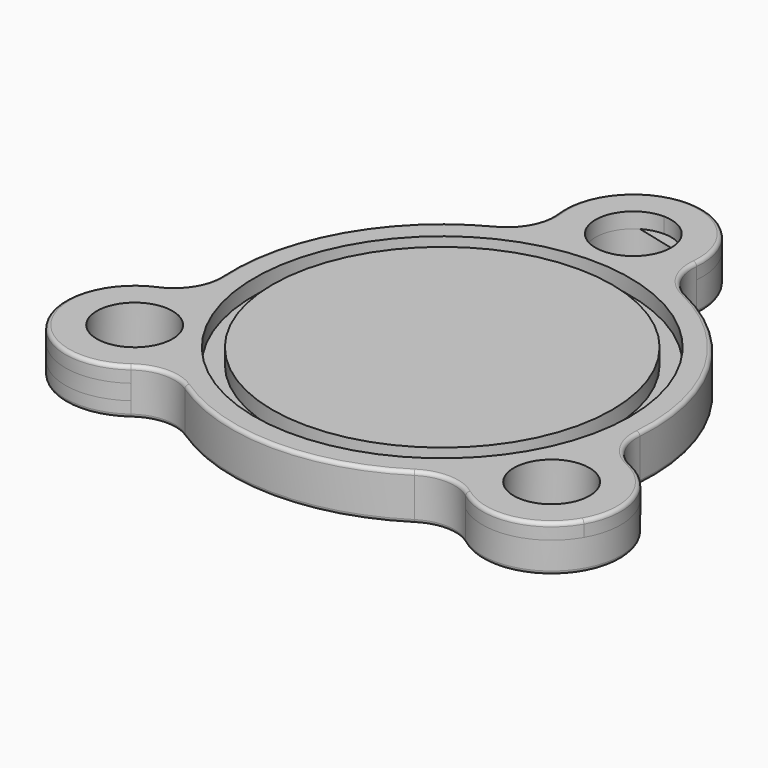
from build123d import *
from build123d import SkipClean  # not in build123d's __all__

# Parameters (mm, degrees)
F0_R     = 23.368
F2_DEPTH = 2.116667
F0_R_2   = 5.207
F0_R_3   = 25.8445
F3_R     = 5.207
F3_R_2   = 25.8445
F4_DEPTH = 2.116667
F5_R     = 5.207
F5_R_2   = 25.8445
F5_R_3   = 23.368
F6_DEPTH = 2.116667
F7_R     = 0.508


# Not quite as in the source:
# - after a boolean that leaves OpenCascade's solid faulty, fix() repairs it


with BuildPart() as f2:
    # F0 (on Top) → F2 (new body)
    with BuildSketch(Plane.XY):
        Circle(F0_R)
    extrude(amount=F2_DEPTH)



with BuildPart() as f2b:
    # F0 (on Top) → F2, piece 2 (new body)
    with BuildSketch(Plane.XY):
        with BuildLine():
            ThreePointArc((9.008634, 32.510164), (6.645647, 39.794521), (-0.316137, 42.984994))
            ThreePointArc((-0.316137, 42.984994), (-7.570395, 39.808854), (-9.915807, 32.245047))
            ThreePointArc((-9.915807, 32.245047), (-10.591058, 28.483521), (-13.302911, 25.790772))
            ThreePointArc((-13.302911, 25.790772), (-25.198767, 14.392829), (-28.972894, -1.644018))
            ThreePointArc((-28.972894, -1.644018), (-29.91458, -5.347837), (-32.811495, -7.840411))
            ThreePointArc((-32.811495, -7.840411), (-37.330955, -21.318933), (-23.425751, -24.275512))
            ThreePointArc((-23.425751, -24.275512), (-19.806913, -23.047075), (-16.138408, -24.118109))
            ThreePointArc((-16.138408, -24.118109), (-0.263504, -29.018304), (15.697768, -24.407201))
            ThreePointArc((15.697768, -24.407201), (19.385118, -23.402963), (22.981051, -24.696914))
            ThreePointArc((22.981051, -24.696914), (30.627799, -26.459145), (37.002427, -21.882867))
            ThreePointArc((37.002427, -21.882867), (37.818424, -14.195745), (32.663705, -8.434966))
            ThreePointArc((32.663705, -8.434966), (29.812532, -5.890196), (28.938261, -2.169887))
            ThreePointArc((28.938261, -2.169887), (25.127534, 14.516832), (12.575213, 26.153306))
            ThreePointArc((12.575213, 26.153306), (9.788992, 28.76903), (9.008634, 32.510164))
        make_face()
        with Locations((-29.059695, -16.595388)):
            Circle(F0_R_2, mode=Mode.SUBTRACT)
        with Locations((28.753535, -17.120367)):
            Circle(F0_R_2, mode=Mode.SUBTRACT)
        Circle(F0_R_3, mode=Mode.SUBTRACT)
        with BuildLine():
            ThreePointArc((4.738233, 33.461217), (-4.180055, 29.80893), (-0.385329, 38.667548))
            ThreePointArc((-0.385329, 38.667548), (3.24252, 37.113503), (4.738233, 33.461217))
        make_face(mode=Mode.SUBTRACT)
    extrude(amount=F2_DEPTH)


with BuildPart() as f2_1:
    add(f2.part, clean=False)

    with SkipClean():  # cleaning this boolean's faces spoils the solid; the shape is the same uncleaned
        add(f2b.part)  # F4 merges F2b
    # F3 (on face) → F4 (join)
    with BuildSketch(Plane(origin=(0, 0, 0), x_dir=(1, 0, 0), z_dir=(0, 0, -1))):
        with BuildLine():
            ThreePointArc((-13.302911, -25.790772), (-10.591058, -28.483521), (-9.915807, -32.245047))
            ThreePointArc((-9.915807, -32.245047), (-0.602192, -42.985282), (9.008634, -32.510164))
            ThreePointArc((9.008634, -32.510164), (9.788992, -28.76903), (12.575213, -26.153306))
            ThreePointArc((12.575213, -26.153306), (25.127534, -14.516832), (28.938261, 2.169887))
            ThreePointArc((28.938261, 2.169887), (29.812532, 5.890196), (32.663705, 8.434966))
            ThreePointArc((32.663705, 8.434966), (36.937653, 21.993337), (22.981051, 24.696914))
            ThreePointArc((22.981051, 24.696914), (19.385118, 23.402963), (15.697768, 24.407201))
            ThreePointArc((15.697768, 24.407201), (-0.263504, 29.018304), (-16.138408, 24.118109))
            ThreePointArc((-16.138408, 24.118109), (-19.806913, 23.047075), (-23.425751, 24.275512))
            ThreePointArc((-23.425751, 24.275512), (-37.330955, 21.318933), (-32.811495, 7.840411))
            ThreePointArc((-32.811495, 7.840411), (-29.91458, 5.347837), (-28.972894, 1.644018))
            ThreePointArc((-28.972894, 1.644018), (-25.198767, -14.392829), (-13.302911, -25.790772))
        make_face()
        with Locations((-0.468767, -33.461217)):
            Circle(F3_R, mode=Mode.SUBTRACT)
        with Locations((-29.059695, 16.595388)):
            Circle(F3_R, mode=Mode.SUBTRACT)
        Circle(F3_R_2, mode=Mode.SUBTRACT)
        with Locations((28.753535, 17.120367)):
            Circle(F3_R, mode=Mode.SUBTRACT)
        Circle(F3_R_2)
    with SkipClean():  # cleaning this boolean's faces spoils the solid; the shape is the same uncleaned
        extrude(amount=F4_DEPTH)

    # F5 (on face) → F6 (join)
    with BuildSketch(Plane(origin=(0, 0, -2.116667), x_dir=(1, 0, 0), z_dir=(0, 0, -1))):
        with BuildLine():
            ThreePointArc((32.663705, 8.434966), (36.937653, 21.993337), (22.981051, 24.696914))
            ThreePointArc((22.981051, 24.696914), (19.385118, 23.402963), (15.697768, 24.407201))
            ThreePointArc((15.697768, 24.407201), (-0.263504, 29.018304), (-16.138408, 24.118109))
            ThreePointArc((-16.138408, 24.118109), (-19.806913, 23.047075), (-23.425751, 24.275512))
            ThreePointArc((-23.425751, 24.275512), (-37.330955, 21.318933), (-32.811495, 7.840411))
            ThreePointArc((-32.811495, 7.840411), (-29.91458, 5.347837), (-28.972894, 1.644018))
            ThreePointArc((-28.972894, 1.644018), (-25.198767, -14.392829), (-13.302911, -25.790772))
            ThreePointArc((-13.302911, -25.790772), (-10.591058, -28.483521), (-9.915807, -32.245047))
            ThreePointArc((-9.915807, -32.245047), (-0.602192, -42.985282), (9.008634, -32.510164))
            ThreePointArc((9.008634, -32.510164), (9.788992, -28.76903), (12.575213, -26.153306))
            ThreePointArc((12.575213, -26.153306), (25.127534, -14.516832), (28.938261, 2.169887))
            ThreePointArc((28.938261, 2.169887), (29.812532, 5.890196), (32.663705, 8.434966))
        make_face()
        with Locations((-0.468767, -33.461217)):
            Circle(F5_R, mode=Mode.SUBTRACT)
        with Locations((-29.059695, 16.595388)):
            Circle(F5_R, mode=Mode.SUBTRACT)
        Circle(F5_R_2, mode=Mode.SUBTRACT)
        with Locations((28.753535, 17.120367)):
            Circle(F5_R, mode=Mode.SUBTRACT)
        Circle(F5_R_3)
    extrude(amount=F6_DEPTH)

    add(f2_1.part.fix(), mode=Mode.REPLACE)

    # F7
    f7_edges = [f2_1.edges().sort_by_distance(p)[0] for p in [
        (9.788992, 28.76903, 2.116667),
        (25.127534, 14.516832, -4.233333),
    ]]
    fillet(f7_edges, radius=F7_R)


solid = f2_1.part
